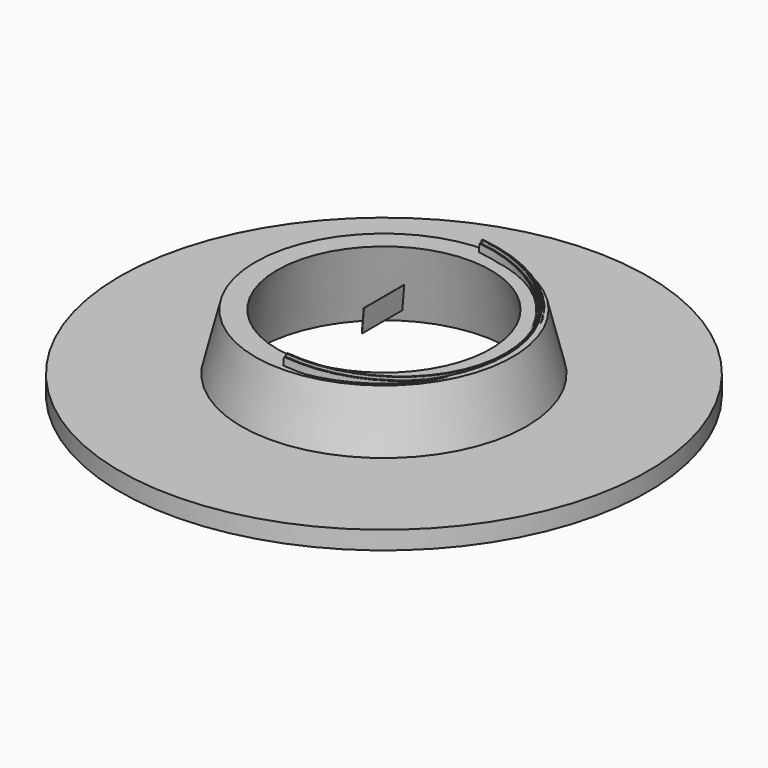
from build123d import *

# Parameters (mm, degrees)
F2_W     = 415.3111577034
F2_H     = 190.7700896263
F3_DEPTH = 2
F4_ANGLE = -5
F6_ANGLE = 179.8


# Not quite as in the source:
# - ends of sketch curves that miss each other by under 0.0002 mm in the source are joined


with BuildPart() as f1:
    # F0 (on Front) → F1 (revolve)
    with BuildSketch(Plane.XZ):
        Polygon((-1176.1225098878, -465.7419486125), (-2176.1225098878, -465.7419486125), (-2176.1225098878, -615.7419486125), (-1033.5217103143, -615.7419486125), (-880, 0), (-1060, 0), align=None)
    revolve(axis=Axis((0, 0, -303.2269775867), (0, 0, -1)))


with BuildPart() as f3:
    # F2 (on Right) → F3 (new body)
    with BuildSketch(Plane.YZ):
        Rectangle(F2_W, F2_H)
    extrude(amount=F3_DEPTH)


with BuildPart() as f3_1:
    # F4: moved
    add(f3.part.rotate(Axis((0, 0, 95.3850448132), (0, -1, 0)), F4_ANGLE))


with BuildPart() as f6:
    # F5 (on face) → F6 (revolve)
    with BuildSketch(Plane(origin=(-6.2893302081, 0, 0.5502450944), x_dir=(0, 1, 0), z_dir=(0.9961946981, 0, -0.0871557427))):
        with BuildLine():
            ThreePointArc((990.31, 67.56), (988.8545963642, 66.0035104881), (987.2040261531, 67.3512780207))
            ThreePointArc((987.2040261531, 67.3512780207), (987.1558886855, 67.4782211989), (987.056723269, 67.5709464659))
            Line((987.056723269, 67.5709464659), (986.89, 67.667204))
            ThreePointArc((986.89, 67.667204), (986.79, 67.840409), (986.889999965, 68.0136140606))
            Line((986.889999965, 68.0136140606), (987.04, 68.100216))
            ThreePointArc((987.04, 68.100216), (987.1498075738, 68.210023918), (987.19, 68.360024))
            Line((987.19, 68.360024), (987.19, 68.720794))
            ThreePointArc((987.19, 68.720794), (987.1498075738, 68.870794082), (987.0399998359, 68.9806017159))
            Line((987.0399998359, 68.9806017159), (986.89, 69.067204))
            ThreePointArc((986.89, 69.067204), (986.79, 69.240409), (986.889999965, 69.4136140606))
            Line((986.889999965, 69.4136140606), (987.04, 69.500216))
            ThreePointArc((987.04, 69.500216), (987.1498075738, 69.610023918), (987.19, 69.760024))
            Line((987.19, 69.760024), (987.19, 70.069992))
            Line((987.19, 70.069992), (986.19, 71.066788))
            Line((986.19, 71.066788), (986.19, 72))
            Line((986.19, 72), (987.19, 72))
            Line((987.19, 72), (987.19, 72.920794))
            ThreePointArc((987.19, 72.920794), (987.1498075738, 73.070794082), (987.0399998359, 73.1806017159))
            Line((987.0399998359, 73.1806017159), (986.89, 73.267204))
            ThreePointArc((986.89, 73.267204), (986.79, 73.440409), (986.889999965, 73.6136140606))
            Line((986.889999965, 73.6136140606), (987.04, 73.700216))
            ThreePointArc((987.04, 73.700216), (987.1498075738, 73.810023918), (987.19, 73.960024))
            Line((987.19, 73.960024), (987.19, 74.320794))
            ThreePointArc((987.19, 74.320794), (987.1498075738, 74.470794082), (987.0399998359, 74.5806017159))
            Line((987.0399998359, 74.5806017159), (986.89, 74.667204))
            ThreePointArc((986.89, 74.667204), (986.79, 74.840409), (986.889999965, 75.0136140606))
            Line((986.889999965, 75.0136140606), (987.04, 75.100216))
            ThreePointArc((987.04, 75.100216), (987.1498075738, 75.210023918), (987.19, 75.360024))
            Line((987.19, 75.360024), (987.19, 76.069992))
            Line((987.19, 76.069992), (986.19, 77.066788))
            Line((986.19, 77.066788), (986.19, 78))
            Line((986.19, 78), (987.19, 78))
            Line((987.19, 78), (987.19, 78.5))
            Line((987.19, 78.5), (986.69, 79))
            Line((986.69, 79), (985.8352329254, 79))
            Line((985.8352329254, 79), (984.2852329254, 79.0000036359))
            Line((984.2852329254, 79.0000036359), (984, 79))
            Line((984, 79), (984, 14.5))
            ThreePointArc((984, 14.5), (984.1464466094, 14.1464466094), (984.5, 14))
            Line((984.5, 14), (1035.5, 14))
            ThreePointArc((1035.5, 14), (1035.8535533906, 14.1464466094), (1036, 14.5))
            Line((1036, 14.5), (1036, 79))
            Line((1036, 79), (1035.7147670746, 79))
            Line((1035.7147670746, 79), (1034.1647670746, 79.0000036359))
            Line((1034.1647670746, 79.0000036359), (1033.31, 79))
            Line((1033.31, 79), (1032.81, 78.5))
            Line((1032.81, 78.5), (1032.81, 78))
            Line((1032.81, 78), (1033.81, 78))
            Line((1033.81, 78), (1033.81, 77.066788))
            Line((1033.81, 77.066788), (1032.81, 76.069992))
            Line((1032.81, 76.069992), (1032.81, 75.360024))
            ThreePointArc((1032.81, 75.360024), (1032.8501924262, 75.210023918), (1032.9600001641, 75.1002162841))
            Line((1032.9600001641, 75.1002162841), (1033.11, 75.013614))
            ThreePointArc((1033.11, 75.013614), (1033.21, 74.840409), (1033.110000035, 74.6672039394))
            Line((1033.110000035, 74.6672039394), (1032.96, 74.580602))
            ThreePointArc((1032.96, 74.580602), (1032.8501924262, 74.470794082), (1032.81, 74.320794))
            Line((1032.81, 74.320794), (1032.81, 73.960024))
            ThreePointArc((1032.81, 73.960024), (1032.8501924262, 73.810023918), (1032.9600001641, 73.7002162841))
            Line((1032.9600001641, 73.7002162841), (1033.11, 73.613614))
            ThreePointArc((1033.11, 73.613614), (1033.21, 73.440409), (1033.110000035, 73.2672039394))
            Line((1033.110000035, 73.2672039394), (1032.96, 73.180602))
            ThreePointArc((1032.96, 73.180602), (1032.8501924262, 73.070794082), (1032.81, 72.920794))
            Line((1032.81, 72.920794), (1032.81, 72))
            Line((1032.81, 72), (1033.81, 72))
            Line((1033.81, 72), (1033.81, 71.066788))
            Line((1033.81, 71.066788), (1032.81, 70.069992))
            Line((1032.81, 70.069992), (1032.81, 69.760024))
            ThreePointArc((1032.81, 69.760024), (1032.8501924262, 69.610023918), (1032.9600001641, 69.5002162841))
            Line((1032.9600001641, 69.5002162841), (1033.11, 69.413614))
            ThreePointArc((1033.11, 69.413614), (1033.21, 69.240409), (1033.110000035, 69.0672039394))
            Line((1033.110000035, 69.0672039394), (1032.96, 68.980602))
            ThreePointArc((1032.96, 68.980602), (1032.8501924262, 68.870794082), (1032.81, 68.720794))
            Line((1032.81, 68.720794), (1032.81, 68.360024))
            ThreePointArc((1032.81, 68.360024), (1032.8501924262, 68.210023918), (1032.9600001641, 68.1002162841))
            Line((1032.9600001641, 68.1002162841), (1033.11, 68.013614))
            ThreePointArc((1033.11, 68.013614), (1033.21, 67.840409), (1033.110000035, 67.6672039394))
            Line((1033.110000035, 67.6672039394), (1032.943276, 67.570946))
            ThreePointArc((1032.943276, 67.570946), (1032.8441103518, 67.4782212544), (1032.7959733699, 67.3512780851))
            ThreePointArc((1032.7959733699, 67.3512780851), (1031.1454036358, 66.0035104881), (1029.69, 67.56))
            Line((1029.69, 67.56), (1029.69, 68.020794))
            ThreePointArc((1029.69, 68.020794), (1029.6498075738, 68.170794082), (1029.5399998359, 68.2806017159))
            Line((1029.5399998359, 68.2806017159), (1029.39, 68.367204))
            ThreePointArc((1029.39, 68.367204), (1029.29, 68.540409), (1029.389999965, 68.7136140606))
            Line((1029.389999965, 68.7136140606), (1029.54, 68.800216))
            ThreePointArc((1029.54, 68.800216), (1029.6498075738, 68.910023918), (1029.69, 69.060024))
            Line((1029.69, 69.060024), (1029.69, 69.420794))
            ThreePointArc((1029.69, 69.420794), (1029.6498075738, 69.570794082), (1029.5399998359, 69.6806017159))
            Line((1029.5399998359, 69.6806017159), (1029.39, 69.767204))
            ThreePointArc((1029.39, 69.767204), (1029.29, 69.940409), (1029.389999965, 70.1136140606))
            Line((1029.389999965, 70.1136140606), (1029.54, 70.200216))
            ThreePointArc((1029.54, 70.200216), (1029.5460502917, 70.2038047453), (1029.5520149457, 70.2075340846))
            Line((1029.5520149457, 70.2075340846), (1028.69, 71.066788))
            Line((1028.69, 71.066788), (1028.69, 72))
            Line((1028.69, 72), (1029.69, 72))
            Line((1029.69, 72), (1029.69, 72.220794))
            ThreePointArc((1029.69, 72.220794), (1029.6498075738, 72.370794082), (1029.5399998359, 72.4806017159))
            Line((1029.5399998359, 72.4806017159), (1029.39, 72.567204))
            ThreePointArc((1029.39, 72.567204), (1029.29, 72.740409), (1029.389999965, 72.9136140606))
            Line((1029.389999965, 72.9136140606), (1029.54, 73.000216))
            ThreePointArc((1029.54, 73.000216), (1029.6498075738, 73.110023918), (1029.69, 73.260024))
            Line((1029.69, 73.260024), (1029.69, 73.620794))
            ThreePointArc((1029.69, 73.620794), (1029.6498075738, 73.770794082), (1029.5399998359, 73.8806017159))
            Line((1029.5399998359, 73.8806017159), (1029.39, 73.967204))
            ThreePointArc((1029.39, 73.967204), (1029.29, 74.140409), (1029.389999965, 74.3136140606))
            Line((1029.389999965, 74.3136140606), (1029.54, 74.400216))
            ThreePointArc((1029.54, 74.400216), (1029.6498075738, 74.510023918), (1029.69, 74.660024))
            Line((1029.69, 74.660024), (1029.69, 75.020794))
            ThreePointArc((1029.69, 75.020794), (1029.6498075738, 75.170794082), (1029.5399998359, 75.2806017159))
            Line((1029.5399998359, 75.2806017159), (1029.39, 75.367204))
            ThreePointArc((1029.39, 75.367204), (1029.29, 75.540409), (1029.389999965, 75.7136140606))
            Line((1029.389999965, 75.7136140606), (1029.54, 75.800216))
            ThreePointArc((1029.54, 75.800216), (1029.6523053421, 75.9144358565), (1029.6898286519, 76.070162022))
            Line((1029.6898286519, 76.070162022), (1028.69, 77.066788))
            Line((1028.69, 77.066788), (1028.69, 78))
            Line((1028.69, 78), (1029.69, 78))
            Line((1029.69, 78), (1029.69, 78.5))
            Line((1029.69, 78.5), (1029.19, 79))
            Line((1029.19, 79), (1026.5, 79))
            Line((1026.5, 79), (1026.5, 67))
            ThreePointArc((1026.5, 67), (1026.2071067812, 66.2928932188), (1025.5, 66))
            Line((1025.5, 66), (1021.05, 66))
            Line((1021.05, 66), (1020.75, 65.7))
            Line((1020.75, 65.7), (1020.45, 66))
            Line((1020.45, 66), (1016, 66))
            ThreePointArc((1016, 66), (1015.2928932188, 66.2928932188), (1015, 67))
            Line((1015, 67), (1015, 96))
            Line((1015, 96), (1013.299999, 96))
            Line((1013.299999, 96), (1012.1, 94.800001))
            Line((1012.1, 94.800001), (1012.1, 93.819615))
            ThreePointArc((1012.1, 93.819615), (1012.1401923012, 93.6696151345), (1012.249999731, 93.5598075341))
            Line((1012.249999731, 93.5598075341), (1012.4, 93.473205))
            ThreePointArc((1012.4, 93.473205), (1012.5, 93.3), (1012.400000035, 93.1267949394))
            Line((1012.400000035, 93.1267949394), (1012.25, 93.040193))
            ThreePointArc((1012.25, 93.040193), (1012.1401924262, 92.930385082), (1012.1, 92.780385))
            Line((1012.1, 92.780385), (1012.1, 92.019615))
            ThreePointArc((1012.1, 92.019615), (1012.1401923012, 91.8696151345), (1012.249999731, 91.7598075341))
            Line((1012.249999731, 91.7598075341), (1012.4, 91.673205))
            ThreePointArc((1012.4, 91.673205), (1012.5, 91.5), (1012.400000035, 91.3267949394))
            Line((1012.400000035, 91.3267949394), (1012.25, 91.240193))
            ThreePointArc((1012.25, 91.240193), (1012.1401924262, 91.130385082), (1012.1, 90.980385))
            Line((1012.1, 90.980385), (1012.1, 90.219615))
            ThreePointArc((1012.1, 90.219615), (1012.1401923012, 90.0696151345), (1012.249999731, 89.9598075341))
            Line((1012.249999731, 89.9598075341), (1012.4, 89.873205))
            ThreePointArc((1012.4, 89.873205), (1012.5, 89.7), (1012.400000035, 89.5267949394))
            Line((1012.400000035, 89.5267949394), (1012.25, 89.440193))
            ThreePointArc((1012.25, 89.440193), (1012.1401924262, 89.330385082), (1012.1, 89.180385))
            Line((1012.1, 89.180385), (1012.1, 88.419615))
            ThreePointArc((1012.1, 88.419615), (1012.1401923012, 88.2696151345), (1012.249999731, 88.1598075341))
            Line((1012.249999731, 88.1598075341), (1012.4, 88.073205))
            ThreePointArc((1012.4, 88.073205), (1012.5, 87.9), (1012.400000035, 87.7267949394))
            Line((1012.400000035, 87.7267949394), (1012.25, 87.640193))
            ThreePointArc((1012.25, 87.640193), (1012.1401924262, 87.530385082), (1012.1, 87.380385))
            Line((1012.1, 87.380385), (1012.1, 86.619615))
            ThreePointArc((1012.1, 86.619615), (1012.1401923012, 86.4696151345), (1012.249999731, 86.3598075341))
            Line((1012.249999731, 86.3598075341), (1012.4, 86.273205))
            ThreePointArc((1012.4, 86.273205), (1012.5, 86.1), (1012.400000035, 85.9267949394))
            Line((1012.400000035, 85.9267949394), (1012.25, 85.840193))
            ThreePointArc((1012.25, 85.840193), (1012.1401924262, 85.730385082), (1012.1, 85.580385))
            Line((1012.1, 85.580385), (1012.1, 84.819615))
            ThreePointArc((1012.1, 84.819615), (1012.1401923012, 84.6696151345), (1012.249999731, 84.5598075341))
            Line((1012.249999731, 84.5598075341), (1012.4, 84.473205))
            ThreePointArc((1012.4, 84.473205), (1012.5, 84.3), (1012.400000035, 84.1267949394))
            Line((1012.400000035, 84.1267949394), (1012.25, 84.040193))
            ThreePointArc((1012.25, 84.040193), (1012.1405353359, 83.930906023), (1012.1000002083, 83.781630999))
            Line((1012.1000002083, 83.781630999), (1012.1, 83.1))
            ThreePointArc((1012.1, 83.1), (1011.6606601718, 82.0393398282), (1010.6, 81.6))
            Line((1010.6, 81.6), (1009.4, 81.6))
            ThreePointArc((1009.4, 81.6), (1008.3393398282, 82.0393398282), (1007.9, 83.1))
            Line((1007.9, 83.1), (1007.899999, 84.680385))
            ThreePointArc((1007.899999, 84.680385), (1007.8598073573, 84.830385457), (1007.7499990859, 84.9401931489))
            Line((1007.7499990859, 84.9401931489), (1007.6, 85.026795))
            ThreePointArc((1007.6, 85.026795), (1007.499999, 85.2), (1007.599999715, 85.3732054936))
            Line((1007.599999715, 85.3732054936), (1007.749999, 85.459808))
            ThreePointArc((1007.749999, 85.459808), (1007.8598074823, 85.5696147595), (1007.9, 85.719615))
            Line((1007.9, 85.719615), (1007.899999, 86.480385))
            ThreePointArc((1007.899999, 86.480385), (1007.8598073573, 86.630385457), (1007.7499990859, 86.7401931489))
            Line((1007.7499990859, 86.7401931489), (1007.6, 86.826795))
            ThreePointArc((1007.6, 86.826795), (1007.499999, 87), (1007.599999715, 87.1732054936))
            Line((1007.599999715, 87.1732054936), (1007.749999, 87.259808))
            ThreePointArc((1007.749999, 87.259808), (1007.8598074823, 87.3696147595), (1007.9, 87.519615))
            Line((1007.9, 87.519615), (1007.899999, 88.280385))
            ThreePointArc((1007.899999, 88.280385), (1007.8598073573, 88.430385457), (1007.7499990859, 88.5401931489))
            Line((1007.7499990859, 88.5401931489), (1007.6, 88.626795))
            ThreePointArc((1007.6, 88.626795), (1007.499999, 88.8), (1007.599999715, 88.9732054936))
            Line((1007.599999715, 88.9732054936), (1007.749999, 89.059808))
            ThreePointArc((1007.749999, 89.059808), (1007.8598074823, 89.1696147595), (1007.9, 89.319615))
            Line((1007.9, 89.319615), (1007.899999, 90.080385))
            ThreePointArc((1007.899999, 90.080385), (1007.8598073573, 90.230385457), (1007.7499990859, 90.3401931489))
            Line((1007.7499990859, 90.3401931489), (1007.6, 90.426795))
            ThreePointArc((1007.6, 90.426795), (1007.499999, 90.6), (1007.599999715, 90.7732054936))
            Line((1007.599999715, 90.7732054936), (1007.749999, 90.859808))
            ThreePointArc((1007.749999, 90.859808), (1007.8598074823, 90.9696147595), (1007.9, 91.119615))
            Line((1007.9, 91.119615), (1007.899999, 91.880385))
            ThreePointArc((1007.899999, 91.880385), (1007.8598073573, 92.030385457), (1007.7499990859, 92.1401931489))
            Line((1007.7499990859, 92.1401931489), (1007.6, 92.226795))
            ThreePointArc((1007.6, 92.226795), (1007.499999, 92.4), (1007.599999715, 92.5732054936))
            Line((1007.599999715, 92.5732054936), (1007.749999, 92.659808))
            ThreePointArc((1007.749999, 92.659808), (1007.8598074823, 92.7696147595), (1007.9, 92.919615))
            Line((1007.9, 92.919615), (1007.899999, 93.680385))
            ThreePointArc((1007.899999, 93.680385), (1007.8598073573, 93.830385457), (1007.7499990859, 93.9401931489))
            Line((1007.7499990859, 93.9401931489), (1007.6, 94.026795))
            ThreePointArc((1007.6, 94.026795), (1007.499999, 94.2), (1007.599999715, 94.3732054936))
            Line((1007.599999715, 94.3732054936), (1007.749999, 94.459808))
            ThreePointArc((1007.749999, 94.459808), (1007.8807367727, 94.6138470255), (1007.8841426572, 94.8158592226))
            Line((1007.8841426572, 94.8158592226), (1006.700001, 96))
            Line((1006.700001, 96), (1005, 96))
            Line((1005, 96), (1005, 67))
            ThreePointArc((1005, 67), (1004.7071067812, 66.2928932188), (1004, 66))
            Line((1004, 66), (999.55, 66))
            Line((999.55, 66), (999.25, 65.7))
            Line((999.25, 65.7), (998.95, 66))
            Line((998.95, 66), (994.5, 66))
            ThreePointArc((994.5, 66), (993.7928932188, 66.2928932188), (993.5, 67))
            Line((993.5, 67), (993.5, 79))
            Line((993.5, 79), (993.1352329254, 79))
            Line((993.1352329254, 79), (991.6352329254, 79.0000036359))
            Line((991.6352329254, 79.0000036359), (990.81, 79))
            Line((990.81, 79), (990.31, 78.5))
            Line((990.31, 78.5), (990.31, 78))
            Line((990.31, 78), (991.31, 78))
            Line((991.31, 78), (991.31, 77.066788))
            Line((991.31, 77.066788), (990.310171, 76.070162))
            ThreePointArc((990.310171, 76.070162), (990.3476946661, 75.9144358417), (990.4600001641, 75.8002162841))
            Line((990.4600001641, 75.8002162841), (990.61, 75.713614))
            ThreePointArc((990.61, 75.713614), (990.71, 75.540409), (990.610000035, 75.3672039394))
            Line((990.610000035, 75.3672039394), (990.46, 75.280602))
            ThreePointArc((990.46, 75.280602), (990.3501924262, 75.170794082), (990.31, 75.020794))
            Line((990.31, 75.020794), (990.31, 74.660024))
            ThreePointArc((990.31, 74.660024), (990.3501924262, 74.510023918), (990.4600001641, 74.4002162841))
            Line((990.4600001641, 74.4002162841), (990.61, 74.313614))
            ThreePointArc((990.61, 74.313614), (990.71, 74.140409), (990.610000035, 73.9672039394))
            Line((990.610000035, 73.9672039394), (990.46, 73.880602))
            ThreePointArc((990.46, 73.880602), (990.3501924262, 73.770794082), (990.31, 73.620794))
            Line((990.31, 73.620794), (990.31, 73.260024))
            ThreePointArc((990.31, 73.260024), (990.3501924262, 73.110023918), (990.4600001641, 73.0002162841))
            Line((990.4600001641, 73.0002162841), (990.61, 72.913614))
            ThreePointArc((990.61, 72.913614), (990.71, 72.740409), (990.610000035, 72.5672039394))
            Line((990.610000035, 72.5672039394), (990.46, 72.480602))
            ThreePointArc((990.46, 72.480602), (990.3501924262, 72.370794082), (990.31, 72.220794))
            Line((990.31, 72.220794), (990.31, 72))
            Line((990.31, 72), (991.31, 72))
            Line((991.31, 72), (991.31, 71.066788))
            Line((991.31, 71.066788), (990.447984, 70.207534))
            ThreePointArc((990.447984, 70.207534), (990.4539493489, 70.2038049642), (990.4600001641, 70.2002162841))
            Line((990.4600001641, 70.2002162841), (990.61, 70.113614))
            ThreePointArc((990.61, 70.113614), (990.71, 69.940409), (990.610000035, 69.7672039394))
            Line((990.610000035, 69.7672039394), (990.46, 69.680602))
            ThreePointArc((990.46, 69.680602), (990.3501924262, 69.570794082), (990.31, 69.420794))
            Line((990.31, 69.420794), (990.31, 69.060024))
            ThreePointArc((990.31, 69.060024), (990.3501924262, 68.910023918), (990.4600001641, 68.8002162841))
            Line((990.4600001641, 68.8002162841), (990.61, 68.713614))
            ThreePointArc((990.61, 68.713614), (990.71, 68.540409), (990.610000035, 68.3672039394))
            Line((990.610000035, 68.3672039394), (990.46, 68.280602))
            ThreePointArc((990.46, 68.280602), (990.3501924262, 68.170794082), (990.31, 68.020794))
            Line((990.31, 68.020794), (990.31, 67.56))
        make_face()
        with BuildLine():
            Line((995.5, 18.5), (986.6, 18.5))
            ThreePointArc((986.6, 18.5), (986.2464466094, 18.6464466094), (986.1, 19))
            Line((986.1, 19), (986.1, 63.2))
            ThreePointArc((986.1, 63.2), (986.2464466094, 63.5535533906), (986.6, 63.7))
            Line((986.6, 63.7), (1033.4, 63.7))
            ThreePointArc((1033.4, 63.7), (1033.7535533906, 63.5535533906), (1033.9, 63.2))
            Line((1033.9, 63.2), (1033.9, 19))
            ThreePointArc((1033.9, 19), (1033.7535533906, 18.6464466094), (1033.4, 18.5))
            Line((1033.4, 18.5), (1024.5, 18.5))
            Line((1024.5, 18.5), (1024.5, 20.2))
            Line((1024.5, 20.2), (1023, 20.2))
            Line((1023, 20.2), (1023, 18.5))
            Line((1023, 18.5), (997, 18.5))
            Line((997, 18.5), (997, 20.2))
            Line((997, 20.2), (995.5, 20.2))
            Line((995.5, 20.2), (995.5, 18.5))
        make_face(mode=Mode.SUBTRACT)
        with BuildLine():
            ThreePointArc((1013, 67), (1012.7071067812, 66.2928932188), (1012, 66))
            Line((1012, 66), (1008, 66))
            ThreePointArc((1008, 66), (1007.2928932188, 66.2928932188), (1007, 67))
            Line((1007, 67), (1007, 78))
            ThreePointArc((1007, 78), (1007.2928932188, 78.7071067812), (1008, 79))
            Line((1008, 79), (1012, 79))
            ThreePointArc((1012, 79), (1012.7071067812, 78.7071067812), (1013, 78))
            Line((1013, 78), (1013, 67))
        make_face(mode=Mode.SUBTRACT)
    revolve(axis=Axis((-2.1484704059, 0, 47.880489211), (-0.0871557427, 0, -0.9961946981)), revolution_arc=F6_ANGLE)


solid = Compound([f1.part, f3_1.part, f6.part])
